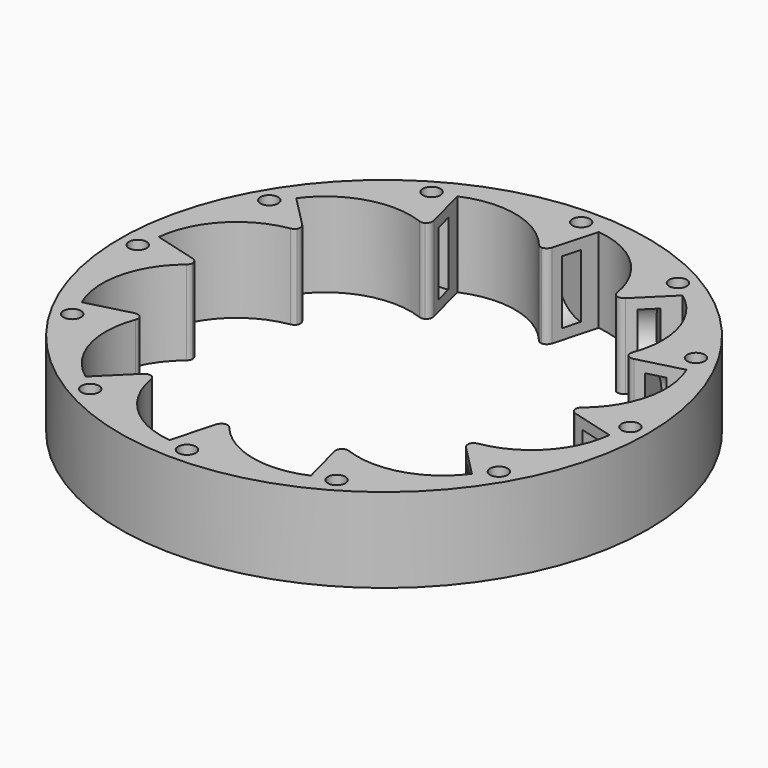
from build123d import *

# Parameters (mm, degrees)
F0_R        = 75
F0_R_2      = 2.5
F1_DEPTH    = 24
F2_T1_DEPTH = 28.7135412507
F2_T3_DEPTH = 31.820725312
F3_W        = 5.2
F3_H        = 9
F5_W        = 5.2
F5_H        = 9
F7_W        = 5.2
F7_H        = 9
F9_W        = 5.2
F9_H        = 9
F11_W       = 5.2
F11_H       = 9
F13_W       = 5.2
F13_H       = 9
F15_W       = 5.2
F15_H       = 9
F17_W       = 5.2
F17_H       = 9
F19_W       = 5.2
F19_H       = 9
F21_W       = 5.2
F21_H       = 9
F23_W       = 5.2
F23_H       = 9
F25_W       = 5.2
F25_H       = 9


# Not quite as in the source:
# - a fillet or chamfer that OpenCascade refuses, or shapes differently, is made with other operations: its cross-section is extruded or revolved along the edge and cut away or added


with BuildPart() as f1:
    # F0 (on Top) → F1 (new body)
    with BuildSketch(Plane.XY):
        Circle(F0_R)
        with Locations((-35, -60.6217782649)):
            Circle(F0_R_2, mode=Mode.SUBTRACT)
        with Locations((-60.6217782649, -35)):
            Circle(F0_R_2, mode=Mode.SUBTRACT)
        with Locations((0, -70)):
            Circle(F0_R_2, mode=Mode.SUBTRACT)
        with Locations((35, -60.6217782649)):
            Circle(F0_R_2, mode=Mode.SUBTRACT)
        with Locations((60.6217782649, -35)):
            Circle(F0_R_2, mode=Mode.SUBTRACT)
        with Locations((-70, 0)):
            Circle(F0_R_2, mode=Mode.SUBTRACT)
        with Locations((-60.6217782649, 35)):
            Circle(F0_R_2, mode=Mode.SUBTRACT)
        with Locations((-35, 60.6217782649)):
            Circle(F0_R_2, mode=Mode.SUBTRACT)
        with BuildLine():
            ThreePointArc((47.6313972081, 27.5), (48.1590007851, 26.5652149131), (48.6682611369, 25.6203114327))
            Line((48.6682611369, 25.6203114327), (62.5386747714, 29.2402626562))
            ThreePointArc((62.5386747714, 29.2402626562), (63.8628004781, 13.3069433392), (55, 0))
            ThreePointArc((55, 0), (54.9895255573, -1.0733494209), (54.9581062189, -2.1462900149))
            Line((54.9581062189, -2.1462900149), (68.7802123992, -5.9465271121))
            ThreePointArc((68.7802123992, -5.9465271121), (61.9602792404, -20.4072492606), (47.6313972081, -27.5))
            ThreePointArc((47.6313972081, -27.5), (47.0856513643, -28.4243106443), (46.521971122, -29.3377947863))
            Line((46.521971122, -29.3377947863), (56.5921476593, -39.539949743))
            ThreePointArc((56.5921476593, -39.539949743), (43.4555512175, -48.6533359013), (27.5, -47.6313972081))
            ThreePointArc((27.5, -47.6313972081), (26.5652149131, -48.1590007851), (25.6203114327, -48.6682611369))
            Line((25.6203114327, -48.6682611369), (29.2402626562, -62.5386747714))
            ThreePointArc((29.2402626562, -62.5386747714), (13.3069433392, -63.8628004781), (0, -55))
            ThreePointArc((0, -55), (-1.0733494209, -54.9895255573), (-2.1462900149, -54.9581062189))
            Line((-2.1462900149, -54.9581062189), (-5.9465271121, -68.7802123992))
            ThreePointArc((-5.9465271121, -68.7802123992), (-20.4072492606, -61.9602792404), (-27.5, -47.6313972081))
            ThreePointArc((-27.5, -47.6313972081), (-28.4243106443, -47.0856513643), (-29.3377947863, -46.521971122))
            Line((-29.3377947863, -46.521971122), (-39.539949743, -56.5921476593))
            ThreePointArc((-39.539949743, -56.5921476593), (-48.6533359013, -43.4555512175), (-47.6313972081, -27.5))
            ThreePointArc((-47.6313972081, -27.5), (-48.1590007851, -26.5652149131), (-48.6682611369, -25.6203114327))
            Line((-48.6682611369, -25.6203114327), (-62.5386747714, -29.2402626562))
            ThreePointArc((-62.5386747714, -29.2402626562), (-63.8628004781, -13.3069433392), (-55, 0))
            ThreePointArc((-55, 0), (-54.9895255573, 1.0733494209), (-54.9581062189, 2.1462900149))
            Line((-54.9581062189, 2.1462900149), (-68.7802123992, 5.9465271121))
            ThreePointArc((-68.7802123992, 5.9465271121), (-61.9602792404, 20.4072492606), (-47.6313972081, 27.5))
            ThreePointArc((-47.6313972081, 27.5), (-47.0856513643, 28.4243106443), (-46.521971122, 29.3377947863))
            Line((-46.521971122, 29.3377947863), (-56.5921476593, 39.539949743))
            ThreePointArc((-56.5921476593, 39.539949743), (-43.4555512175, 48.6533359013), (-27.5, 47.6313972081))
            ThreePointArc((-27.5, 47.6313972081), (-26.5652149131, 48.1590007851), (-25.6203114327, 48.6682611369))
            Line((-25.6203114327, 48.6682611369), (-29.2402626562, 62.5386747714))
            ThreePointArc((-29.2402626562, 62.5386747714), (-13.3069433392, 63.8628004781), (0, 55))
            ThreePointArc((0, 55), (1.0733494209, 54.9895255573), (2.1462900149, 54.9581062189))
            Line((2.1462900149, 54.9581062189), (5.9465271121, 68.7802123992))
            ThreePointArc((5.9465271121, 68.7802123992), (20.4072492606, 61.9602792404), (27.5, 47.6313972081))
            ThreePointArc((27.5, 47.6313972081), (28.4243106443, 47.0856513643), (29.3377947863, 46.521971122))
            Line((29.3377947863, 46.521971122), (39.539949743, 56.5921476593))
            ThreePointArc((39.539949743, 56.5921476593), (48.6533359013, 43.4555512175), (47.6313972081, 27.5))
        make_face(mode=Mode.SUBTRACT)
        with Locations((70, 0)):
            Circle(F0_R_2, mode=Mode.SUBTRACT)
        with Locations((60.6217782649, 35)):
            Circle(F0_R_2, mode=Mode.SUBTRACT)
        with Locations((0, 70)):
            Circle(F0_R_2, mode=Mode.SUBTRACT)
        with Locations((35, 60.6217782649)):
            Circle(F0_R_2, mode=Mode.SUBTRACT)
    extrude(amount=F1_DEPTH)

    # F2: fillet of radius 2 on 24 edges, made by hand

    # F2_s2 → F2_t1 (cut)
    with BuildSketch(Plane.XY.offset(-2.3567706253)):
        with BuildLine():
            ThreePointArc((48.5444127172, -27.3681843784), (47.7446967943, -27.6869420566), (47.1530637041, -28.3123397711))
            ThreePointArc((47.1530637041, -28.3123397711), (47.3939709413, -27.9071947429), (47.6313972081, -27.5))
            ThreePointArc((47.6313972081, -27.5), (48.0885305527, -27.4384253126), (48.5444127172, -27.3681843784))
        make_face()
        with BuildLine():
            ThreePointArc((55.7247868141, 0.5706634314), (55.1915913481, -0.105246777), (54.9919209196, -0.9426736303))
            ThreePointArc((54.9919209196, -0.9426736303), (54.9979801928, -0.4713541251), (55, 0))
            ThreePointArc((55, 0), (55.3651017456, 0.2818919158), (55.7247868141, 0.5706634314))
        make_face()
        with BuildLine():
            ThreePointArc((47.9737492858, 28.3566024357), (47.8499435712, 27.5046492916), (48.0957373344, 26.6795811484))
            ThreePointArc((48.0957373344, 26.6795811484), (47.8653250663, 27.0907854499), (47.6313972081, 27.5))
            ThreePointArc((47.6313972081, 27.5), (47.8066386369, 27.926676433), (47.9737492858, 28.3566024357))
        make_face()
        with BuildLine():
            ThreePointArc((27.3681843784, 48.5444127172), (27.6869420566, 47.7446967943), (28.3123397711, 47.1530637041))
            ThreePointArc((28.3123397711, 47.1530637041), (27.9071947429, 47.3939709413), (27.5, 47.6313972081))
            ThreePointArc((27.5, 47.6313972081), (27.4384253126, 48.0885305527), (27.3681843784, 48.5444127172))
        make_face()
        with BuildLine():
            ThreePointArc((-0.5706634314, 55.7247868141), (0.105246777, 55.1915913481), (0.9426736303, 54.9919209196))
            ThreePointArc((0.9426736303, 54.9919209196), (0.4713541251, 54.9979801928), (0, 55))
            ThreePointArc((0, 55), (-0.2818919158, 55.3651017456), (-0.5706634314, 55.7247868141))
        make_face()
        with BuildLine():
            ThreePointArc((-28.3566024357, 47.9737492858), (-27.5046492916, 47.8499435712), (-26.6795811484, 48.0957373344))
            ThreePointArc((-26.6795811484, 48.0957373344), (-27.0907854499, 47.8653250663), (-27.5, 47.6313972081))
            ThreePointArc((-27.5, 47.6313972081), (-27.926676433, 47.8066386369), (-28.3566024357, 47.9737492858))
        make_face()
        with BuildLine():
            ThreePointArc((-48.5444127172, 27.3681843784), (-47.7446967943, 27.6869420566), (-47.1530637041, 28.3123397711))
            ThreePointArc((-47.1530637041, 28.3123397711), (-47.3939709413, 27.9071947429), (-47.6313972081, 27.5))
            ThreePointArc((-47.6313972081, 27.5), (-48.0885305527, 27.4384253126), (-48.5444127172, 27.3681843784))
        make_face()
        with BuildLine():
            ThreePointArc((28.3566024357, -47.9737492858), (27.5046492916, -47.8499435712), (26.6795811484, -48.0957373344))
            ThreePointArc((26.6795811484, -48.0957373344), (27.0907854499, -47.8653250663), (27.5, -47.6313972081))
            ThreePointArc((27.5, -47.6313972081), (27.926676433, -47.8066386369), (28.3566024357, -47.9737492858))
        make_face()
        with BuildLine():
            ThreePointArc((0.5706634314, -55.7247868141), (-0.105246777, -55.1915913481), (-0.9426736303, -54.9919209196))
            ThreePointArc((-0.9426736303, -54.9919209196), (-0.4713541251, -54.9979801928), (0, -55))
            ThreePointArc((0, -55), (0.2818919158, -55.3651017456), (0.5706634314, -55.7247868141))
        make_face()
        with BuildLine():
            ThreePointArc((-27.3681843784, -48.5444127172), (-27.6869420566, -47.7446967943), (-28.3123397711, -47.1530637041))
            ThreePointArc((-28.3123397711, -47.1530637041), (-27.9071947429, -47.3939709413), (-27.5, -47.6313972081))
            ThreePointArc((-27.5, -47.6313972081), (-27.4384253126, -48.0885305527), (-27.3681843784, -48.5444127172))
        make_face()
        with BuildLine():
            ThreePointArc((-47.9737492858, -28.3566024357), (-47.8499435712, -27.5046492916), (-48.0957373344, -26.6795811484))
            ThreePointArc((-48.0957373344, -26.6795811484), (-47.8653250663, -27.0907854499), (-47.6313972081, -27.5))
            ThreePointArc((-47.6313972081, -27.5), (-47.8066386369, -27.926676433), (-47.9737492858, -28.3566024357))
        make_face()
        with BuildLine():
            ThreePointArc((-55.7247868141, -0.5706634314), (-55.1915913481, 0.105246777), (-54.9919209196, 0.9426736303))
            ThreePointArc((-54.9919209196, 0.9426736303), (-54.9979801928, 0.4713541251), (-55, 0))
            ThreePointArc((-55, 0), (-55.3651017456, -0.2818919158), (-55.7247868141, -0.5706634314))
        make_face()
    extrude(amount=F2_T1_DEPTH, mode=Mode.SUBTRACT)

    # F2_s4 → F2_t3 (cut)
    with BuildSketch(Plane.XY.offset(-3.910362656)):
        with BuildLine():
            ThreePointArc((47.3233077029, -28.0268540521), (47.0590442233, -29.2895984831), (47.6207649404, -30.450989253))
            Line((47.6207649404, -30.450989253), (46.521971122, -29.3377947863))
            ThreePointArc((46.521971122, -29.3377947863), (46.9272173779, -28.6851227846), (47.3233077029, -28.0268540521))
        make_face()
        with BuildLine():
            ThreePointArc((54.9966136879, -0.6103137458), (55.3991270167, -1.8360142413), (56.4662868126, -2.5609477933))
            Line((56.4662868126, -2.5609477933), (54.9581062189, -2.1462900149))
            ThreePointArc((54.9581062189, -2.1462900149), (54.9827237705, -1.3784363531), (54.9966136879, -0.6103137458))
        make_face()
        with BuildLine():
            ThreePointArc((47.9336214487, 26.9697596358), (48.8950584646, 26.1095285337), (50.1817127337, 26.0152975595))
            Line((50.1817127337, 26.0152975595), (48.6682611369, 25.6203114327))
            ThreePointArc((48.6682611369, 25.6203114327), (48.3056537311, 26.2976009859), (47.9336214487, 26.9697596358))
        make_face()
        with BuildLine():
            ThreePointArc((28.0268540521, 47.3233077029), (29.2895984831, 47.0590442233), (30.450989253, 47.6207649404))
            Line((30.450989253, 47.6207649404), (29.3377947863, 46.521971122))
            ThreePointArc((29.3377947863, 46.521971122), (28.6851227846, 46.9272173779), (28.0268540521, 47.3233077029))
        make_face()
        with BuildLine():
            ThreePointArc((0.6103137458, 54.9966136879), (1.8360142413, 55.3991270167), (2.5609477933, 56.4662868126))
            Line((2.5609477933, 56.4662868126), (2.1462900149, 54.9581062189))
            ThreePointArc((2.1462900149, 54.9581062189), (1.3784363531, 54.9827237705), (0.6103137458, 54.9966136879))
        make_face()
        with BuildLine():
            ThreePointArc((-26.9697596358, 47.9336214487), (-26.1095285337, 48.8950584646), (-26.0152975595, 50.1817127337))
            Line((-26.0152975595, 50.1817127337), (-25.6203114327, 48.6682611369))
            ThreePointArc((-25.6203114327, 48.6682611369), (-26.2976009859, 48.3056537311), (-26.9697596358, 47.9336214487))
        make_face()
        with BuildLine():
            ThreePointArc((-47.3233077029, 28.0268540521), (-47.0590442233, 29.2895984831), (-47.6207649404, 30.450989253))
            Line((-47.6207649404, 30.450989253), (-46.521971122, 29.3377947863))
            ThreePointArc((-46.521971122, 29.3377947863), (-46.9272173779, 28.6851227846), (-47.3233077029, 28.0268540521))
        make_face()
        with BuildLine():
            ThreePointArc((26.9697596358, -47.9336214487), (26.1095285337, -48.8950584646), (26.0152975595, -50.1817127337))
            Line((26.0152975595, -50.1817127337), (25.6203114327, -48.6682611369))
            ThreePointArc((25.6203114327, -48.6682611369), (26.2976009859, -48.3056537311), (26.9697596358, -47.9336214487))
        make_face()
        with BuildLine():
            ThreePointArc((-2.5609477933, -56.4662868126), (-1.8360142413, -55.3991270167), (-0.6103137458, -54.9966136879))
            ThreePointArc((-0.6103137458, -54.9966136879), (-1.3784363531, -54.9827237705), (-2.1462900149, -54.9581062189))
            Line((-2.1462900149, -54.9581062189), (-2.5609477933, -56.4662868126))
        make_face()
        with BuildLine():
            ThreePointArc((-28.0268540521, -47.3233077029), (-29.2895984831, -47.0590442233), (-30.450989253, -47.6207649404))
            Line((-30.450989253, -47.6207649404), (-29.3377947863, -46.521971122))
            ThreePointArc((-29.3377947863, -46.521971122), (-28.6851227846, -46.9272173779), (-28.0268540521, -47.3233077029))
        make_face()
        with BuildLine():
            ThreePointArc((-47.9336214487, -26.9697596358), (-48.8950584646, -26.1095285337), (-50.1817127337, -26.0152975595))
            Line((-50.1817127337, -26.0152975595), (-48.6682611369, -25.6203114327))
            ThreePointArc((-48.6682611369, -25.6203114327), (-48.3056537311, -26.2976009859), (-47.9336214487, -26.9697596358))
        make_face()
        with BuildLine():
            ThreePointArc((-54.9966136879, 0.6103137458), (-55.3991270167, 1.8360142413), (-56.4662868126, 2.5609477933))
            Line((-56.4662868126, 2.5609477933), (-54.9581062189, 2.1462900149))
            ThreePointArc((-54.9581062189, 2.1462900149), (-54.9827237705, 1.3784363531), (-54.9966136879, 0.6103137458))
        make_face()
    extrude(amount=F2_T3_DEPTH, mode=Mode.SUBTRACT)

    # F3 (on face) → F4 (revolve, cut)
    with BuildSketch(Plane(origin=(-3.1565656566, 12.0948788029, 0), x_dir=(0.9675903042, 0.2525252525, 0), z_dir=(0.2525252525, -0.9675903042, 0))):
        with Locations((60.3957200593, 16.5)):
            Rectangle(F3_W, F3_H)
    revolve(axis=Axis((55.2817474897, 27.3463232623, 12), (-0.9675903042, -0.2525252525, 0)), mode=Mode.SUBTRACT)

    # F5 (on face) → F6 (revolve, cut)
    with BuildSketch(Plane(origin=(3.3137733541, 12.0527551273, 0), x_dir=(0.9642204102, -0.2651018683, 0), z_dir=(-0.2651018683, -0.9642204102, 0))):
        with Locations((60.3957200593, 16.5)):
            Rectangle(F5_W, F5_H)
    revolve(axis=Axis((61.5485593228, -3.9582630996, 12), (-0.9642204102, 0.2651018683, 0)), mode=Mode.SUBTRACT)

    # F7 (on face) → F8 (revolve, cut)
    with BuildSketch(Plane(origin=(8.8961894707, 8.7811054487, 0), x_dir=(0.7024884359, -0.7116951577, 0), z_dir=(-0.7116951577, -0.7024884359, 0))):
        with Locations((60.3957200593, 16.5)):
            Rectangle(F7_W, F7_H)
    revolve(axis=Axis((51.3234843901, -34.2022360606, 12), (-0.7024884359, 0.7116951577, 0)), mode=Mode.SUBTRACT)

    # F9 (on face) → F10 (revolve, cut)
    with BuildSketch(Plane(origin=(12.0948788029, 3.1565656566, 0), x_dir=(0.2525252525, -0.9675903042, 0), z_dir=(-0.9675903042, -0.2525252525, 0))):
        with Locations((60.3957200593, 16.5)):
            Rectangle(F9_W, F9_H)
    revolve(axis=Axis((27.3463232623, -55.2817474897, 12), (-0.2525252525, 0.9675903042, 0)), mode=Mode.SUBTRACT)

    # F11 (on face) → F12 (revolve, cut)
    with BuildSketch(Plane(origin=(12.0527551273, -3.3137733541, 0), x_dir=(-0.2651018683, -0.9642204102, 0), z_dir=(-0.9642204102, 0.2651018683, 0))):
        with Locations((60.3957200593, 16.5)):
            Rectangle(F11_W, F11_H)
    revolve(axis=Axis((-3.9582630996, -61.5485593228, 12), (0.2651018683, 0.9642204102, 0)), mode=Mode.SUBTRACT)

    # F13 (on face) → F14 (revolve, cut)
    with BuildSketch(Plane(origin=(8.7811054487, -8.8961894707, 0), x_dir=(-0.7116951577, -0.7024884359, 0), z_dir=(-0.7024884359, 0.7116951577, 0))):
        with Locations((60.3957200593, 16.5)):
            Rectangle(F13_W, F13_H)
    revolve(axis=Axis((-34.2022360606, -51.3234843901, 12), (0.7116951577, 0.7024884359, 0)), mode=Mode.SUBTRACT)

    # F15 (on face) → F16 (revolve, cut)
    with BuildSketch(Plane(origin=(3.1565656566, -12.0948788029, 0), x_dir=(-0.9675903042, -0.2525252525, 0), z_dir=(-0.2525252525, 0.9675903042, 0))):
        with Locations((60.3957200593, 16.5)):
            Rectangle(F15_W, F15_H)
    revolve(axis=Axis((-55.2817474897, -27.3463232623, 12), (0.9675903042, 0.2525252525, 0)), mode=Mode.SUBTRACT)

    # F17 (on face) → F18 (revolve, cut)
    with BuildSketch(Plane(origin=(-3.3137733541, -12.0527551273, 0), x_dir=(-0.9642204102, 0.2651018683, 0), z_dir=(0.2651018683, 0.9642204102, 0))):
        with Locations((60.3957200593, 16.5)):
            Rectangle(F17_W, F17_H)
    revolve(axis=Axis((-61.5485593228, 3.9582630996, 12), (0.9642204102, -0.2651018683, 0)), mode=Mode.SUBTRACT)

    # F19 (on face) → F20 (revolve, cut)
    with BuildSketch(Plane(origin=(-8.8961894707, -8.7811054487, 0), x_dir=(-0.7024884359, 0.7116951577, 0), z_dir=(0.7116951577, 0.7024884359, 0))):
        with Locations((60.3957200593, 16.5)):
            Rectangle(F19_W, F19_H)
    revolve(axis=Axis((-51.3234843901, 34.2022360606, 12), (0.7024884359, -0.7116951577, 0)), mode=Mode.SUBTRACT)

    # F21 (on face) → F22 (revolve, cut)
    with BuildSketch(Plane(origin=(-12.0948788029, -3.1565656566, 0), x_dir=(-0.2525252525, 0.9675903042, 0), z_dir=(0.9675903042, 0.2525252525, 0))):
        with Locations((60.3957200593, 16.5)):
            Rectangle(F21_W, F21_H)
    revolve(axis=Axis((-27.3463232623, 55.2817474897, 12), (0.2525252525, -0.9675903042, 0)), mode=Mode.SUBTRACT)

    # F23 (on face) → F24 (revolve, cut)
    with BuildSketch(Plane(origin=(-12.0527551273, 3.3137733541, 0), x_dir=(0.2651018683, 0.9642204102, 0), z_dir=(0.9642204102, -0.2651018683, 0))):
        with Locations((60.3957200593, 16.5)):
            Rectangle(F23_W, F23_H)
    revolve(axis=Axis((3.9582630996, 61.5485593228, 12), (-0.2651018683, -0.9642204102, 0)), mode=Mode.SUBTRACT)

    # F25 (on face) → F26 (revolve, cut)
    with BuildSketch(Plane(origin=(-8.7811054487, 8.8961894707, 0), x_dir=(0.7116951577, 0.7024884359, 0), z_dir=(0.7024884359, -0.7116951577, 0))):
        with Locations((60.3957200593, 16.5)):
            Rectangle(F25_W, F25_H)
    revolve(axis=Axis((34.2022360606, 51.3234843901, 12), (-0.7116951577, -0.7024884359, 0)), mode=Mode.SUBTRACT)


solid = f1.part
